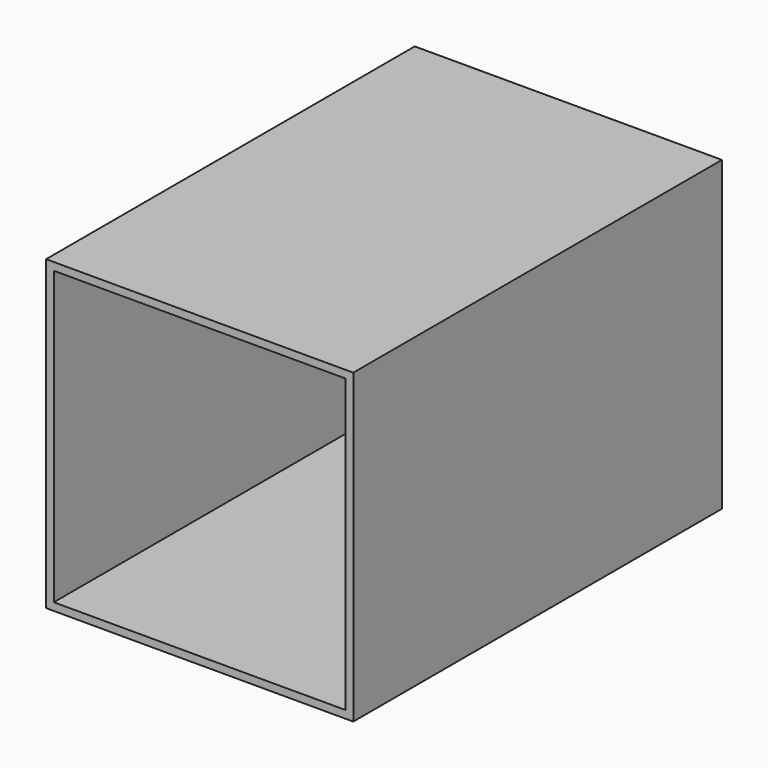
from build123d import *

# Parameters (mm, degrees)
F1_DEPTH = 25
F0_W     = 200
F0_H     = 200
F2_DEPTH = 25
F3_DEPTH = 275


with BuildPart() as f1:
    # F0 (on Front) → F1 (new body)
    with BuildSketch(Plane.XZ):
        with BuildLine():
            Line((80.3527337313, 115.043669641), (-14.6472653884, 115.043669641))
            ThreePointArc((-14.6472653884, 115.043669641), (52.5278782552, 87.2188135425), (80.3527337313, 20.043669641))
            Line((80.3527337313, 20.043669641), (80.3527337313, 115.043669641))
        make_face()
    extrude(amount=F1_DEPTH)


with BuildPart() as f1b:
    # F0 (on Front) → F1, piece 2 (new body)
    with BuildSketch(Plane.XZ):
        with BuildLine():
            Line((-14.6472653884, 115.043669641), (-109.6472662687, 115.043669641))
            Line((-109.6472662687, 115.043669641), (-109.6472662687, 20.0436696216))
            ThreePointArc((-109.6472662687, 20.0436696216), (-81.8224101771, 87.2188141581), (-14.6472653884, 115.043669641))
        make_face()
    extrude(amount=F1_DEPTH)


with BuildPart() as f1c:
    # F0 (on Front) → F1, piece 3 (new body)
    with BuildSketch(Plane.XZ):
        with BuildLine():
            ThreePointArc((-14.6472666457, -74.956330359), (-81.8224106079, -47.1314744453), (-109.6472662687, 20.0436696216))
            Line((-109.6472662687, 20.0436696216), (-109.6472662687, -74.956330359))
            Line((-109.6472662687, -74.956330359), (-14.6472666457, -74.956330359))
        make_face()
    extrude(amount=F1_DEPTH)


with BuildPart() as f1d:
    # F0 (on Front) → F1, piece 4 (new body)
    with BuildSketch(Plane.XZ):
        with BuildLine():
            Line((80.3527337313, -74.956330359), (80.3527337313, 20.043669641))
            ThreePointArc((80.3527337313, 20.043669641), (52.5278778107, -47.131474705), (-14.6472666457, -74.956330359))
            Line((-14.6472666457, -74.956330359), (80.3527337313, -74.956330359))
        make_face()
    extrude(amount=F1_DEPTH)


with BuildPart() as f2:
    # F0 (on Front) → F2 (new body)
    with BuildSketch(Plane.XZ):
        with Locations((-14.6472662687, 20.043669641)):
            Rectangle(F0_W, F0_H)
        Polygon((-109.6472662687, 20.0436696216), (-109.6472662687, 115.043669641), (-14.6472653884, 115.043669641), (80.3527337313, 115.043669641), (80.3527337313, 20.043669641), (80.3527337313, -74.956330359), (-14.6472666457, -74.956330359), (-109.6472662687, -74.956330359), align=None, mode=Mode.SUBTRACT)
    extrude(amount=F2_DEPTH)

    # F3 (add): a face of the model
    f3_faces = [f2.faces().sort_by_distance(p)[0] for p in [
        (-14.6472662687, -25, 117.2152425163),
    ]]
    extrude(f3_faces, amount=F3_DEPTH)


solid = Compound([f1.part, f1b.part, f1c.part, f1d.part, f2.part])
